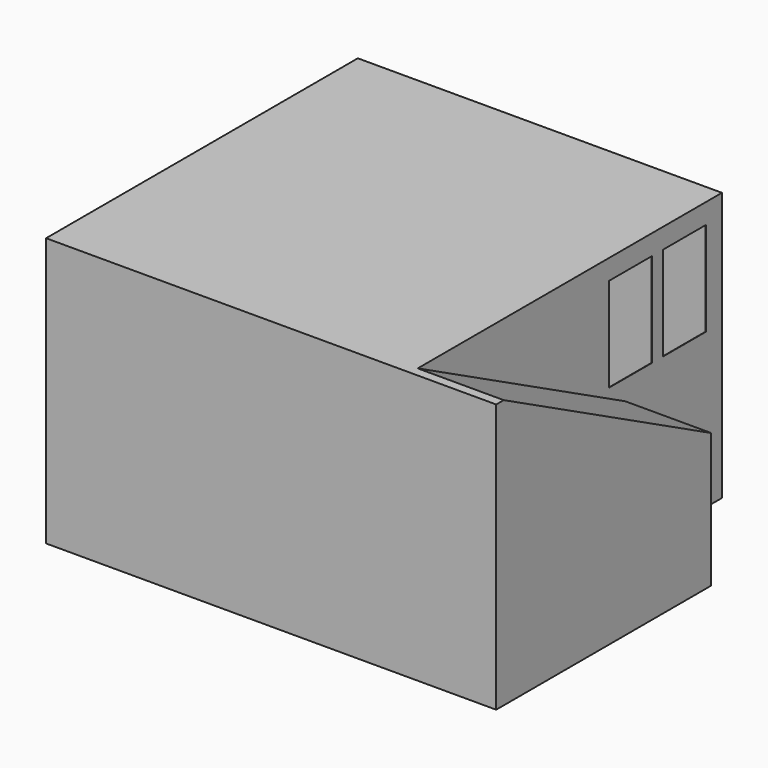
from build123d import *

# Parameters (mm, degrees)
F0_W      = 3350
F0_H      = 2900
F1_DEPTH  = 2000
F5_DEPTH  = 640
F9_DEPTH  = 2900
F10_T     = -2.5
F11_W     = 400
F11_H     = 700
F12_DEPTH = 2.5


# Not quite as in the source:
# - an extrude ends at something that could not be found from the text; its depth is read off the source's solid
# - a feature of the source that left no trace in its solid (it failed there, or was rolled back) is left out


with BuildPart() as f1:
    # F0 (on Top) → F1 (new body)
    with BuildSketch(Plane.XY):
        with Locations((1675, 1460.2979007226)):
            Rectangle(F0_W, F0_H)
    extrude(amount=F1_DEPTH)

    # F4 (on face) → F5 (cut, through all)
    with BuildSketch(Plane.YZ.offset(3350)):
        Polygon((2910.2979007226, 2000), (80.2979007226, 2000), (2010.2979007226, 1000), (2010.2979007226, 0), (2910.2979007226, 0), (2910.2979007226, 1000), align=None)
    extrude(amount=-F5_DEPTH, mode=Mode.SUBTRACT)

    # F8 (on face) → F9 (join, through all)
    with BuildSketch(Plane(origin=(0, 2910.2979007226, 0), x_dir=(-1, 0, 0), z_dir=(0, 1, 0))):
        Polygon((-2310, 1000), (-1030, 2000), (-2710, 2000), (-2710, 0), (-2310, 0), align=None)
    extrude(amount=-F9_DEPTH)

    # F10
    f10_openings = [f1.faces().sort_by_distance(p)[0] for p in [
        (1589.598971, 1397.271311, 0),
    ]]
    offset(amount=F10_T, openings=f10_openings, kind=Kind.INTERSECTION)

    # F11 (on face) → F12 (cut, through all)
    with BuildSketch(Plane.YZ.offset(2710)):
        with Locations((2560.2979007226, 1500)):
            Rectangle(F11_W, F11_H)
        with Locations((2060.2979007226, 1500)):
            Rectangle(F11_W, F11_H)
    extrude(amount=-F12_DEPTH, mode=Mode.SUBTRACT)


solid = f1.part
